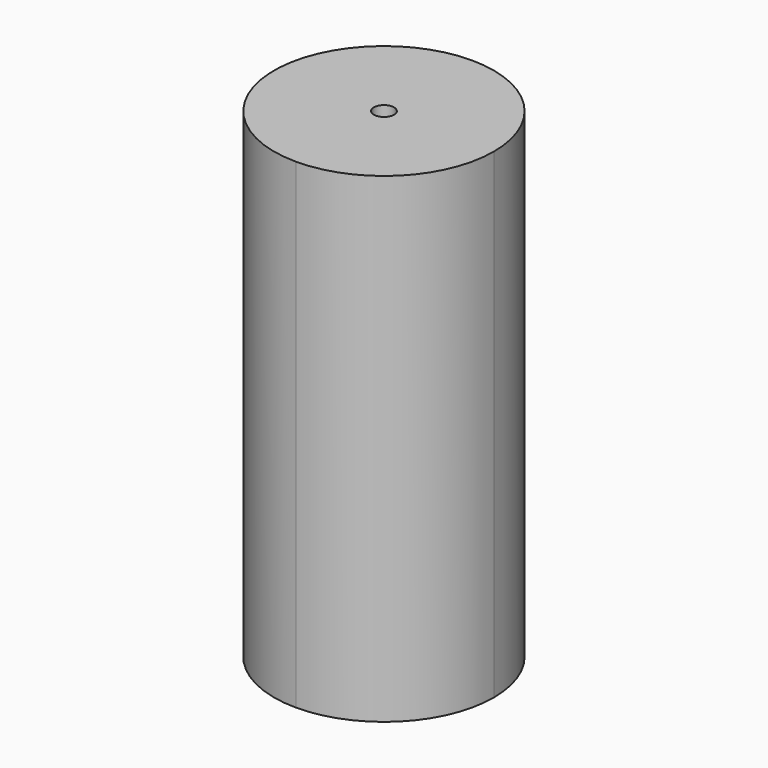
from build123d import *

# Parameters (mm, degrees)
F1_DEPTH = 1
F2_DEPTH = 85
F3_START = 85
F3_DEPTH = 20
F4_START = 60
F4_DEPTH = 20
F6_D     = 4.4
F6_DEPTH = 19
F6_TIP   = 1.321893
F7_D     = 3
F7_DEPTH = 6
F7_TIP   = 0.901291


with BuildPart() as f1:
    # F0 (on Top) → F1 (new body)
    with BuildSketch(Plane.XY):
        with BuildLine():
            ThreePointArc((-1.438285, -18.945483), (-19, 0), (-1.438285, 18.945483))
            ThreePointArc((-1.438285, 18.945483), (-0.719659, 18.986366), (0, 19))
            Line((0, 19), (0, 24))
            ThreePointArc((0, 24), (-24, 0), (0, -24))
            Line((0, -24), (0, -19))
            ThreePointArc((0, -19), (-0.719659, -18.986366), (-1.438285, -18.945483))
        make_face()
        with BuildLine():
            ThreePointArc((0, 19), (0.719659, 18.986366), (1.438285, 18.945483))
            ThreePointArc((1.438285, 18.945483), (13.934264, 12.916512), (19, 0))
            ThreePointArc((19, 0), (13.934264, -12.916512), (1.438285, -18.945483))
            ThreePointArc((1.438285, -18.945483), (0.719659, -18.986366), (0, -19))
            Line((0, -19), (0, -24))
            ThreePointArc((0, -24), (16.970563, -16.970563), (24, 0))
            ThreePointArc((24, 0), (16.970563, 16.970563), (0, 24))
            Line((0, 24), (0, 19))
        make_face()
    extrude(amount=F1_DEPTH)

    # F0 (on Top) → F2 (join)
    with BuildSketch(Plane.XY):
        with BuildLine():
            ThreePointArc((0, 19), (0.719659, 18.986366), (1.438285, 18.945483))
            ThreePointArc((1.438285, 18.945483), (13.934264, 12.916512), (19, 0))
            ThreePointArc((19, 0), (13.934264, -12.916512), (1.438285, -18.945483))
            ThreePointArc((1.438285, -18.945483), (0.719659, -18.986366), (0, -19))
            Line((0, -19), (0, -24))
            ThreePointArc((0, -24), (16.970563, -16.970563), (24, 0))
            ThreePointArc((24, 0), (16.970563, 16.970563), (0, 24))
            Line((0, 24), (0, 19))
        make_face()
        with BuildLine():
            ThreePointArc((-1.438285, -18.945483), (-19, 0), (-1.438285, 18.945483))
            ThreePointArc((-1.438285, 18.945483), (-0.719659, 18.986366), (0, 19))
            Line((0, 19), (0, 24))
            ThreePointArc((0, 24), (-24, 0), (0, -24))
            Line((0, -24), (0, -19))
            ThreePointArc((0, -19), (-0.719659, -18.986366), (-1.438285, -18.945483))
        make_face()
    extrude(amount=F2_DEPTH)

    # F0 (on Top) → F3 (join)
    with BuildSketch(Plane.XY.offset(F3_START)):
        with BuildLine():
            ThreePointArc((14.870984, -3.378808), (15.15495, -1.7), (15.25, 0))
            ThreePointArc((15.25, 0), (15.15495, 1.7), (14.870984, 3.378808))
            ThreePointArc((14.870984, 3.378808), (10.066133, 11.455805), (1.438285, 15.182023))
            Line((1.438285, 15.182023), (1.438285, 12.870561))
            Line((1.438285, 12.870561), (0, 12.870561))
            Line((0, 12.870561), (-1.438285, 12.870561))
            Line((-1.438285, 12.870561), (-1.438285, 15.182023))
            ThreePointArc((-1.438285, 15.182023), (-10.066133, 11.455805), (-14.870984, 3.378808))
            ThreePointArc((-14.870984, 3.378808), (-15.25, 0), (-14.870984, -3.378808))
            ThreePointArc((-14.870984, -3.378808), (-10.066133, -11.455805), (-1.438285, -15.182023))
            Line((-1.438285, -15.182023), (-1.438285, -12.870561))
            Line((-1.438285, -12.870561), (0, -12.870561))
            Line((0, -12.870561), (1.438285, -12.870561))
            Line((1.438285, -12.870561), (1.438285, -15.182023))
            ThreePointArc((1.438285, -15.182023), (10.066133, -11.455805), (14.870984, -3.378808))
        make_face()
        with BuildLine():
            ThreePointArc((-14.870984, -3.378808), (-15.25, 0), (-14.870984, 3.378808))
            ThreePointArc((-14.870984, 3.378808), (-18.65, 0), (-14.870984, -3.378808))
        make_face()
        with BuildLine():
            ThreePointArc((1.438285, 15.182023), (10.066133, 11.455805), (14.870984, 3.378808))
            ThreePointArc((14.870984, 3.378808), (18.65, 0), (14.870984, -3.378808))
            ThreePointArc((14.870984, -3.378808), (10.066133, -11.455805), (1.438285, -15.182023))
            Line((1.438285, -15.182023), (1.438285, -18.945483))
            ThreePointArc((1.438285, -18.945483), (13.934264, -12.916512), (19, 0))
            ThreePointArc((19, 0), (13.934264, 12.916512), (1.438285, 18.945483))
            Line((1.438285, 18.945483), (1.438285, 15.182023))
        make_face()
        with BuildLine():
            ThreePointArc((0, 19), (0.719659, 18.986366), (1.438285, 18.945483))
            ThreePointArc((1.438285, 18.945483), (13.934264, 12.916512), (19, 0))
            ThreePointArc((19, 0), (13.934264, -12.916512), (1.438285, -18.945483))
            ThreePointArc((1.438285, -18.945483), (0.719659, -18.986366), (0, -19))
            Line((0, -19), (0, -24))
            ThreePointArc((0, -24), (16.970563, -16.970563), (24, 0))
            ThreePointArc((24, 0), (16.970563, 16.970563), (0, 24))
            Line((0, 24), (0, 19))
        make_face()
        with BuildLine():
            ThreePointArc((-1.438285, -18.945483), (-19, 0), (-1.438285, 18.945483))
            ThreePointArc((-1.438285, 18.945483), (-0.719659, 18.986366), (0, 19))
            Line((0, 19), (0, 24))
            ThreePointArc((0, 24), (-24, 0), (0, -24))
            Line((0, -24), (0, -19))
            ThreePointArc((0, -19), (-0.719659, -18.986366), (-1.438285, -18.945483))
        make_face()
        with BuildLine():
            ThreePointArc((14.870984, 3.378808), (15.15495, 1.7), (15.25, 0))
            ThreePointArc((15.25, 0), (15.15495, -1.7), (14.870984, -3.378808))
            ThreePointArc((14.870984, -3.378808), (18.65, 0), (14.870984, 3.378808))
        make_face()
        with BuildLine():
            ThreePointArc((-14.870984, 3.378808), (-10.066133, 11.455805), (-1.438285, 15.182023))
            Line((-1.438285, 15.182023), (-1.438285, 18.945483))
            ThreePointArc((-1.438285, 18.945483), (-19, 0), (-1.438285, -18.945483))
            Line((-1.438285, -18.945483), (-1.438285, -15.182023))
            ThreePointArc((-1.438285, -15.182023), (-10.066133, -11.455805), (-14.870984, -3.378808))
            ThreePointArc((-14.870984, -3.378808), (-18.65, 0), (-14.870984, 3.378808))
        make_face()
        with BuildLine():
            ThreePointArc((-1.438285, -15.182023), (0, -15.25), (1.438285, -15.182023))
            Line((1.438285, -15.182023), (1.438285, -12.870561))
            Line((1.438285, -12.870561), (0, -12.870561))
            Line((0, -12.870561), (-1.438285, -12.870561))
            Line((-1.438285, -12.870561), (-1.438285, -15.182023))
        make_face()
        with BuildLine():
            Line((1.438285, -18.945483), (1.438285, -15.182023))
            ThreePointArc((1.438285, -15.182023), (0, -15.25), (-1.438285, -15.182023))
            Line((-1.438285, -15.182023), (-1.438285, -18.945483))
            ThreePointArc((-1.438285, -18.945483), (-0.719659, -18.986366), (0, -19))
            ThreePointArc((0, -19), (0.719659, -18.986366), (1.438285, -18.945483))
        make_face()
        with BuildLine():
            ThreePointArc((-1.438285, 15.182023), (0, 15.25), (1.438285, 15.182023))
            Line((1.438285, 15.182023), (1.438285, 18.945483))
            ThreePointArc((1.438285, 18.945483), (0.719659, 18.986366), (0, 19))
            ThreePointArc((0, 19), (-0.719659, 18.986366), (-1.438285, 18.945483))
            Line((-1.438285, 18.945483), (-1.438285, 15.182023))
        make_face()
        with BuildLine():
            Line((1.438285, 12.870561), (1.438285, 15.182023))
            ThreePointArc((1.438285, 15.182023), (0, 15.25), (-1.438285, 15.182023))
            Line((-1.438285, 15.182023), (-1.438285, 12.870561))
            Line((-1.438285, 12.870561), (0, 12.870561))
            Line((0, 12.870561), (1.438285, 12.870561))
        make_face()
    extrude(amount=F3_DEPTH)

    # F0 (on Top) → F4 (join)
    with BuildSketch(Plane.XY.offset(F4_START)):
        with BuildLine():
            ThreePointArc((-1.438285, -15.182023), (0, -15.25), (1.438285, -15.182023))
            Line((1.438285, -15.182023), (1.438285, -12.870561))
            Line((1.438285, -12.870561), (0, -12.870561))
            Line((0, -12.870561), (-1.438285, -12.870561))
            Line((-1.438285, -12.870561), (-1.438285, -15.182023))
        make_face()
        with BuildLine():
            Line((1.438285, -18.945483), (1.438285, -15.182023))
            ThreePointArc((1.438285, -15.182023), (0, -15.25), (-1.438285, -15.182023))
            Line((-1.438285, -15.182023), (-1.438285, -18.945483))
            ThreePointArc((-1.438285, -18.945483), (-0.719659, -18.986366), (0, -19))
            ThreePointArc((0, -19), (0.719659, -18.986366), (1.438285, -18.945483))
        make_face()
        with BuildLine():
            Line((1.438285, 12.870561), (1.438285, 15.182023))
            ThreePointArc((1.438285, 15.182023), (0, 15.25), (-1.438285, 15.182023))
            Line((-1.438285, 15.182023), (-1.438285, 12.870561))
            Line((-1.438285, 12.870561), (0, 12.870561))
            Line((0, 12.870561), (1.438285, 12.870561))
        make_face()
        with BuildLine():
            ThreePointArc((-1.438285, 15.182023), (0, 15.25), (1.438285, 15.182023))
            Line((1.438285, 15.182023), (1.438285, 18.945483))
            ThreePointArc((1.438285, 18.945483), (0.719659, 18.986366), (0, 19))
            ThreePointArc((0, 19), (-0.719659, 18.986366), (-1.438285, 18.945483))
            Line((-1.438285, 18.945483), (-1.438285, 15.182023))
        make_face()
    extrude(amount=F4_DEPTH)

    # F6
    with Locations(Plane.XY.offset(105)):
        with Locations((0, 0)):
            Hole(F6_D / 2, depth=F6_DEPTH)
            with Locations((0, 0, -(F6_DEPTH + F6_TIP / 2))):  # 118° drill point
                Cone(0, F6_D / 2, F6_TIP, mode=Mode.SUBTRACT)

    # F7
    with Locations(Plane(origin=(0, 0, 0), x_dir=(1, 0, 0), z_dir=(0, 0, -1))):
        with Locations((0, 21.472742), (0, -21.5)):
            Hole(F7_D / 2, depth=F7_DEPTH)
            with Locations((0, 0, -(F7_DEPTH + F7_TIP / 2))):  # 118° drill point
                Cone(0, F7_D / 2, F7_TIP, mode=Mode.SUBTRACT)


solid = f1.part
